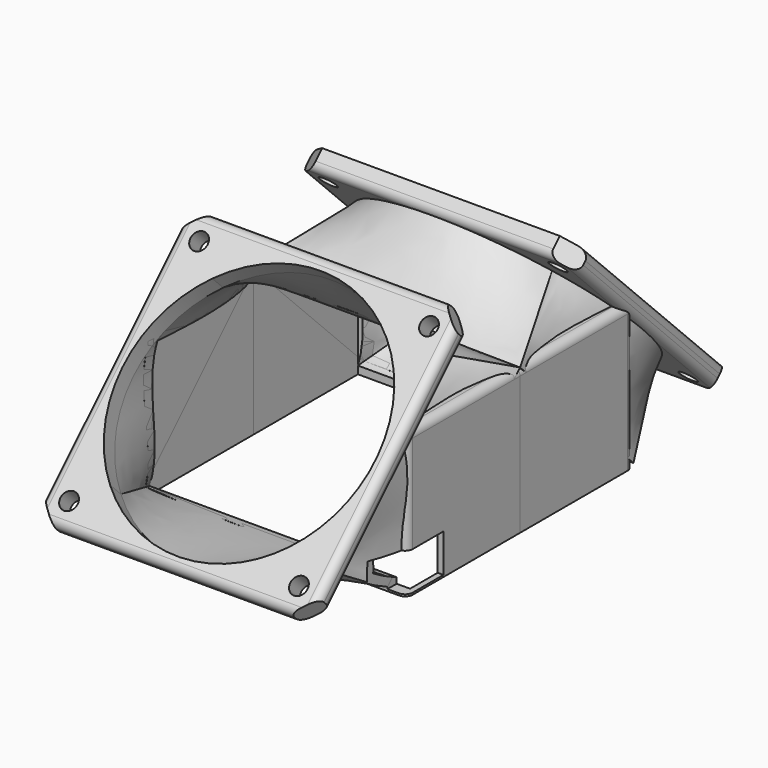
from build123d import *

# Parameters (mm, degrees)
F0_W       = 68
F0_H       = 36
F1_DEPTH   = 34
F5_W       = 68
F5_H       = 48.0832611207
F10_W      = 71
F10_H      = 38
F11_DEPTH  = 37
F17_R      = 2.25
F18_DEPTH  = 5
F13_W      = 71
F13_H      = 52.3259018078
F15_W      = 72
F15_H      = 72
F20_DEPTH  = 5
F22_ANGLE  = 180
F23_ANGLE  = 180
F24_ANGLE  = 180
F25_SIZE   = 5
F25_2_SIZE = 5
F26_R      = 2
F26_2_R    = 2
F26_3_R    = 2
F26_4_R    = 2
F27_W      = 20
F27_H      = 10
F28_DEPTH  = 5


# Not quite as in the source:
# - the arcs of a loft's sections are written as splines that run evenly, so that the points pair up as in the source's solid


with BuildPart() as f1:
    # F0 (on Front) → F1 (new body)
    with BuildSketch(Plane.XZ):
        Rectangle(F0_W, F0_H)
    extrude(amount=F1_DEPTH)


with BuildPart() as f8:
    # F5 (on line) → F8 section 0
    with BuildSketch(Plane(origin=(0, -9, 9), x_dir=(-1, 0, 0), z_dir=(0, 0.7071067812, -0.7071067812))):
        with Locations((0, -11.313708499)):
            Rectangle(F5_W, F5_H)
    # F7 (on offset) → F8 section 1
    with BuildSketch(Plane(origin=(0, -26.3553390593, 26.3553390593), x_dir=(-1, 0, 0), z_dir=(0, 0.7071067812, -0.7071067812))):
        with BuildLine():
            ThreePointArc((22.7247922722, -43.9281008939), (32.9995314428, -20.1752310162), (22.9785256862, 3.6857944454))
            ThreePointArc((22.9785256862, 3.6857944454), (0.9058576713, 12.9881874253), (-21.6440594101, 4.9111565309))
            ThreePointArc((-21.6440594101, 4.9111565309), (-32.9745636064, -18.7039410223), (-23.5316027072, -43.1351433515))
            ThreePointArc((-23.5316027072, -43.1351433515), (-0.5656245977, -52.9945294316), (22.7247922722, -43.9281008939))
        make_face()
    loft()


with BuildPart() as f11:
    # F10 (on face) → F11 (new body)
    with BuildSketch(Plane.XZ):
        with Locations((0, 1)):
            Rectangle(F10_W, F10_H)
    extrude(amount=F11_DEPTH)


with BuildPart() as f18:
    # F8_face (on face) + F17 (on offset) → F18 (new body)
    with BuildSketch(Plane(origin=(0, -40.4970343181, 12.2136438005), x_dir=(1, 0, 0), z_dir=(0, -0.7071067812, 0.7071067812))):
        with BuildLine():
            ThreePointArc((-22.7247922722, -23.928723664), (0.5656245977, -32.9951522017), (23.5316027072, -23.1357661216))
            ThreePointArc((23.5316027072, -23.1357661216), (32.9745636064, 1.2954362076), (21.6440594101, 24.9105337609))
            ThreePointArc((21.6440594101, 24.9105337609), (-0.9058576713, 32.9875646552), (-22.9785256862, 23.6851716753))
            ThreePointArc((-22.9785256862, 23.6851716753), (-32.9995314428, -0.1758537863), (-22.7247922722, -23.928723664))
        make_face()
    with BuildSketch(Plane(origin=(0, -26.3553390593, 26.3553390593), x_dir=(-1, 0, 0), z_dir=(0, 0.7071067812, -0.7071067812))):
        with Locations((30, 10.0006227701)):
            Circle(F17_R)
        with Locations((-30, 10.0006227701)):
            Circle(F17_R)
        with Locations((-30, -49.9993772299)):
            Circle(F17_R)
        with Locations((30, -49.9993772299)):
            Circle(F17_R)
    extrude(amount=F18_DEPTH, dir=(0, -0.7071067812, 0.7071067812))


with BuildPart() as f19:
    # F13 (on line) → F19 section 0
    with BuildSketch(Plane(origin=(0, -10, 10), x_dir=(1, 0, 0), z_dir=(0, -0.7071067812, 0.7071067812))):
        with Locations((0, -12.0208152802)):
            Rectangle(F13_W, F13_H)
    # F14 (on offset) → F19 section 1
    with BuildSketch(Plane(origin=(0, -26.3553390593, 26.3553390593), x_dir=(-1, 0, 0), z_dir=(0, 0.7071067812, -0.7071067812))):
        with BuildLine():
            add(Edge.make_bspline(
                [(25.2267083163, 4.2619744951), (23.6388065591, 5.9130586934), (21.8883304872, 7.4077112602), (18.129328051, 10.0268608868), (16.1208946354, 11.151293183), (11.9231496329, 12.9867715882), (9.7339418435, 13.6977723114), (5.258771261, 14.6790430894), (2.9729191253, 14.9492888805), (-1.6076987413, 15.0386423456), (-3.9023512076, 14.8577478104), (-8.4123857826, 14.0517501591), (-10.627656372, 13.4266669731), (-14.893789556, 11.7562922431), (-16.9445466621, 10.7110420026), (-20.8028333493, 8.2404817581), (-22.6102675266, 6.8152328436), (-24.261351725, 5.2273310864)],
                knots=[0, 0, 0, 0, 0.125, 0.125, 0.25, 0.25, 0.375, 0.375, 0.5, 0.5, 0.625, 0.625, 0.75, 0.75, 0.875, 0.875, 1, 1, 1, 1], degree=3))
            add(Edge.make_bspline(
                [(-24.261351725, 5.2273310864), (-25.9124359233, 3.6394293292), (-27.4070884901, 1.8889532573), (-30.0262381167, -1.8700491789), (-31.1506704129, -3.8784825945), (-32.9861488181, -8.076227597), (-33.6971495413, -10.2654353865), (-34.6784203193, -14.7406059689), (-34.9486661104, -17.0264581046), (-35.0380195756, -21.6070759713), (-34.8571250403, -23.9017284375), (-34.051127389, -28.4117630125), (-33.426044203, -30.6270336019), (-31.7556694731, -34.8931667859), (-30.7104192325, -36.943923892), (-28.239858988, -40.8022105792), (-26.8146100735, -42.6096447565), (-25.2267083163, -44.2607289549)],
                knots=[0, 0, 0, 0, 0.125, 0.125, 0.25, 0.25, 0.375, 0.375, 0.5, 0.5, 0.625, 0.625, 0.75, 0.75, 0.875, 0.875, 1, 1, 1, 1], degree=3))
            add(Edge.make_bspline(
                [(-25.2267083163, -44.2607289549), (-23.6388065591, -45.9118131532), (-21.8883304872, -47.40646572), (-18.129328051, -50.0256153466), (-16.1208946354, -51.1500476428), (-11.9231496329, -52.9855260481), (-9.7339418435, -53.6965267712), (-5.258771261, -54.6777975493), (-2.9729191253, -54.9480433403), (1.6076987413, -55.0373968055), (3.9023512076, -54.8565022702), (8.4123857826, -54.050504619), (10.627656372, -53.4254214329), (14.893789556, -51.755046703), (16.9445466621, -50.7097964624), (20.8028333493, -48.2392362179), (22.6102675266, -46.8139873034), (24.261351725, -45.2260855462)],
                knots=[0, 0, 0, 0, 0.125, 0.125, 0.25, 0.25, 0.375, 0.375, 0.5, 0.5, 0.625, 0.625, 0.75, 0.75, 0.875, 0.875, 1, 1, 1, 1], degree=3))
            add(Edge.make_bspline(
                [(24.261351725, -45.2260855462), (25.9124359233, -43.638183789), (27.4070884901, -41.8877077171), (30.0262381167, -38.1287052809), (31.1506704129, -36.1202718653), (32.9861488181, -31.9225268628), (33.6971495413, -29.7333190734), (34.6784203193, -25.2581484909), (34.9486661104, -22.9722963552), (35.0380195756, -18.3916784886), (34.8571250403, -16.0970260224), (34.051127389, -11.5869914473), (33.426044203, -9.3717208579), (31.7556694731, -5.1055876739), (30.7104192325, -3.0548305678), (28.239858988, 0.8034561194), (26.8146100735, 2.6108902967), (25.2267083163, 4.2619744951)],
                knots=[0, 0, 0, 0, 0.125, 0.125, 0.25, 0.25, 0.375, 0.375, 0.5, 0.5, 0.625, 0.625, 0.75, 0.75, 0.875, 0.875, 1, 1, 1, 1], degree=3))
        make_face()
    loft(ruled=True)

    # F21: cut F18, F8, F1
    add(f18.part, mode=Mode.SUBTRACT)
    add(f8.part, mode=Mode.SUBTRACT)
    add(f1.part, mode=Mode.SUBTRACT)


with BuildPart() as f20:
    # F15 (on offset) → F20 (new body)
    with BuildSketch(Plane(origin=(0, -26.3553390593, 26.3553390593), x_dir=(-1, 0, 0), z_dir=(0, 0.7071067812, -0.7071067812))):
        with Locations((0, -19.9993772299)):
            Rectangle(F15_W, F15_H)
    extrude(amount=-F20_DEPTH)

    # F21: cut F18, F8, F1
    add(f18.part, mode=Mode.SUBTRACT)
    add(f8.part, mode=Mode.SUBTRACT)
    add(f1.part, mode=Mode.SUBTRACT)


with BuildPart() as f11_1:
    add(f11.part)

    # F21: cut F18, F8, F1
    add(f18.part, mode=Mode.SUBTRACT)
    add(f8.part, mode=Mode.SUBTRACT)
    add(f1.part, mode=Mode.SUBTRACT)


with BuildPart() as f22_1:
    # F22: copy of F11
    add(f11_1.part.rotate(Axis((0, 0, 0), (0, 0, -1)), F22_ANGLE))

    # F26#3
    f26_3_edges = [f22_1.edges().sort_by_distance(p)[0] for p in [
        (35.5, 18.5, 20),
        (33.760485, 37, 20),
        (35.5, 37, 1),
        (-35.5, 37, 1),
        (-33.760485, 37, 20),
        (-35.5, 18.5, 20),
    ]]
    fillet(f26_3_edges, radius=F26_3_R)


with BuildPart() as f23_1:
    # F23: copy of F19
    add(f19.part.rotate(Axis((0, 0, 0), (0, 0, -1)), F23_ANGLE))


with BuildPart() as f24_1:
    # F24: copy of F20
    add(f20.part.rotate(Axis((0, 0, 0), (0, 0, -1)), F24_ANGLE))

    # F25#2
    f25_2_edges = [f24_1.edges().sort_by_distance(p)[0] for p in [
        (-36, 16.808957, 39.437255),
        (36, 16.808957, 39.437255),
        (-36, 67.720645, -11.474433),
        (36, 67.720645, -11.474433),
    ]]
    chamfer(f25_2_edges, length=F25_2_SIZE)

    # F26#4
    f26_4_edges = [f24_1.edges().sort_by_distance(p)[0] for p in [
        (36, 44.032568, 15.749178),
        (36, 40.497034, 12.213644),
        (0, 15.04119, 37.669488),
        (0, 65.952878, -13.2422),
        (0, 69.488412, -9.706666),
        (-36, 44.032568, 15.749178),
        (-36, 40.497034, 12.213644),
    ]]
    fillet(f26_4_edges, radius=F26_4_R)


with BuildPart() as f20_1:
    add(f20.part)

    # F25
    f25_edges = [f20_1.edges().sort_by_distance(p)[0] for p in [
        (36, -67.720645, -11.474433),
        (-36, -67.720645, -11.474433),
        (36, -16.808957, 39.437255),
        (-36, -16.808957, 39.437255),
    ]]
    chamfer(f25_edges, length=F25_SIZE)

    # F26#2
    f26_2_edges = [f20_1.edges().sort_by_distance(p)[0] for p in [
        (36, -44.032568, 15.749178),
        (0, -18.576724, 41.205022),
        (-36, -44.032568, 15.749178),
        (0, -69.488412, -9.706666),
        (36, -40.497034, 12.213644),
        (0, -65.952878, -13.2422),
        (-36, -40.497034, 12.213644),
        (0, -15.04119, 37.669488),
    ]]
    fillet(f26_2_edges, radius=F26_2_R)


with BuildPart() as f11_2:
    add(f11_1.part)

    # F26
    f26_edges = [f11_2.edges().sort_by_distance(p)[0] for p in [
        (-35.5, -37, 1),
        (-33.760485, -37, 20),
        (-35.5, -18.5, 20),
        (35.5, -37, 1),
        (35.5, -18.5, 20),
        (33.760485, -37, 20),
    ]]
    fillet(f26_edges, radius=F26_R)


with BuildPart() as f28:
    # F27 (on face) → F28 (new body)
    with BuildSketch(Plane.YZ.offset(35.5)):
        with Locations((-35, -12.5)):
            Rectangle(F27_W, F27_H)
    extrude(amount=-F28_DEPTH)


with BuildPart() as f11_3:
    add(f11_2.part)

    # F29: cut F28
    add(f28.part, mode=Mode.SUBTRACT)


with BuildPart() as f19_1:
    add(f19.part)

    # F29: cut F28
    add(f28.part, mode=Mode.SUBTRACT)


solid = Compound([f22_1.part, f23_1.part, f24_1.part, f20_1.part, f11_3.part, f19_1.part])
